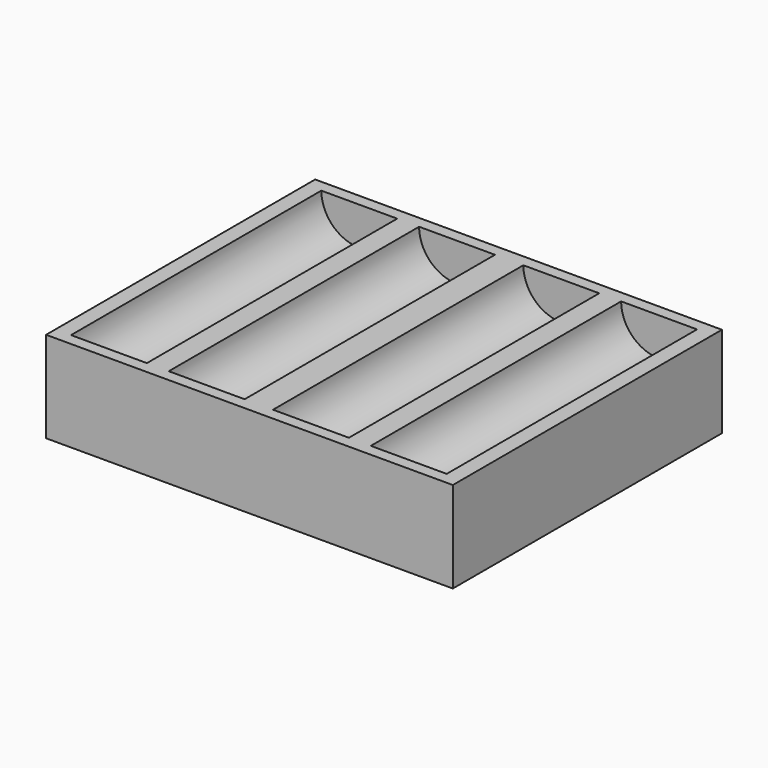
from build123d import *

# Parameters (mm, degrees)
F0_W     = 132.08
F0_H     = 101.6
F1_DEPTH = 17.272
F3_DEPTH = 101.6
F6_DEPTH = 3.81


with BuildPart() as f1:
    # F0 (on Top) → F1 (new body)
    with BuildSketch(Plane.XY):
        with Locations((22.4865525961, 18.1711361257)):
            Rectangle(F0_W, F0_H)
    extrude(amount=F1_DEPTH)

    # F2 (on face) → F3 (join, through all)
    with BuildSketch(Plane.XZ.offset(32.6288638743)):
        with BuildLine():
            Line((-6.7586990196, 29.591), (-13.8706990196, 29.591))
            ThreePointArc((-13.8706990196, 29.591), (-17.4788505821, 20.8801515626), (-26.1896990196, 17.272))
            Line((-26.1896990196, 17.272), (5.560301017, 17.272))
            ThreePointArc((5.560301017, 17.272), (-3.1505474441, 20.8801515496), (-6.7586990196, 29.591))
        make_face()
        with BuildLine():
            ThreePointArc((-26.1896990196, 17.272), (-34.900547457, 20.8801515626), (-38.5086990196, 29.591))
            Line((-38.5086990196, 29.591), (-43.5534474039, 29.591))
            Line((-43.5534474039, 29.591), (-43.5534474039, 17.272))
            Line((-43.5534474039, 17.272), (-26.1896990196, 17.272))
        make_face()
        with BuildLine():
            ThreePointArc((17.8793009804, 29.591), (14.2711494308, 20.8801515755), (5.560301017, 17.272))
            Line((5.560301017, 17.272), (39.4128042118, 17.272))
            ThreePointArc((39.4128042118, 17.272), (30.7019557743, 20.8801515626), (27.0938042118, 29.591))
            Line((27.0938042118, 29.591), (17.8793009804, 29.591))
        make_face()
        with BuildLine():
            ThreePointArc((51.7318042118, 29.591), (48.1236526492, 20.8801515626), (39.4128042118, 17.272))
            Line((39.4128042118, 17.272), (71.1628042118, 17.272))
            ThreePointArc((71.1628042118, 17.272), (62.4519557743, 20.8801515626), (58.8438042118, 29.591))
            Line((58.8438042118, 29.591), (51.7318042118, 29.591))
        make_face()
        with BuildLine():
            ThreePointArc((83.4818042118, 29.591), (79.8736526492, 20.8801515626), (71.1628042118, 17.272))
            Line((71.1628042118, 17.272), (88.5265525961, 17.272))
            Line((88.5265525961, 17.272), (88.5265525961, 29.591))
            Line((88.5265525961, 29.591), (83.4818042118, 29.591))
        make_face()
    extrude(amount=-F3_DEPTH)

    # F5 (on face) → F6 (join)
    with BuildSketch(Plane.XZ.offset(32.6288638743)):
        with BuildLine():
            Line((-43.5534474039, 0), (88.5265525961, 0))
            Line((88.5265525961, 0), (88.5265525961, 29.591))
            Line((88.5265525961, 29.591), (83.4818042118, 29.591))
            ThreePointArc((83.4818042118, 29.591), (71.1628042118, 17.272), (58.8438042118, 29.591))
            Line((58.8438042118, 29.591), (51.7318042118, 29.591))
            ThreePointArc((51.7318042118, 29.591), (39.4128042118, 17.272), (27.0938042118, 29.591))
            Line((27.0938042118, 29.591), (17.8793009804, 29.591))
            ThreePointArc((17.8793009804, 29.591), (5.5603009804, 17.272), (-6.7586990196, 29.591))
            Line((-6.7586990196, 29.591), (-13.8706990196, 29.591))
            ThreePointArc((-13.8706990196, 29.591), (-26.1896990196, 17.272), (-38.5086990196, 29.591))
            Line((-38.5086990196, 29.591), (-43.5534474039, 29.591))
            Line((-43.5534474039, 29.591), (-43.5534474039, 0))
        make_face()
        with BuildLine():
            ThreePointArc((58.8438042118, 29.591), (71.1628042118, 17.272), (83.4818042118, 29.591))
            Line((83.4818042118, 29.591), (58.8438042118, 29.591))
        make_face()
        with BuildLine():
            Line((-13.8706990196, 29.591), (-38.5086990196, 29.591))
            ThreePointArc((-38.5086990196, 29.591), (-26.1896990196, 17.272), (-13.8706990196, 29.591))
        make_face()
        with BuildLine():
            ThreePointArc((27.0938042118, 29.591), (39.4128042118, 17.272), (51.7318042118, 29.591))
            Line((51.7318042118, 29.591), (27.0938042118, 29.591))
        make_face()
        with BuildLine():
            Line((17.8793009804, 29.591), (-6.7586990196, 29.591))
            ThreePointArc((-6.7586990196, 29.591), (5.5603009804, 17.272), (17.8793009804, 29.591))
        make_face()
    extrude(amount=F6_DEPTH)

    # F7: F1 across plane


with BuildPart() as f1_1:
    add(f1.part)
    add(f1.part.mirror(Plane(origin=(22.4865525961, 18.1711361257, 11.7082126405), x_dir=(1, 0, 0), z_dir=(0, -1, 0))))


solid = f1_1.part
